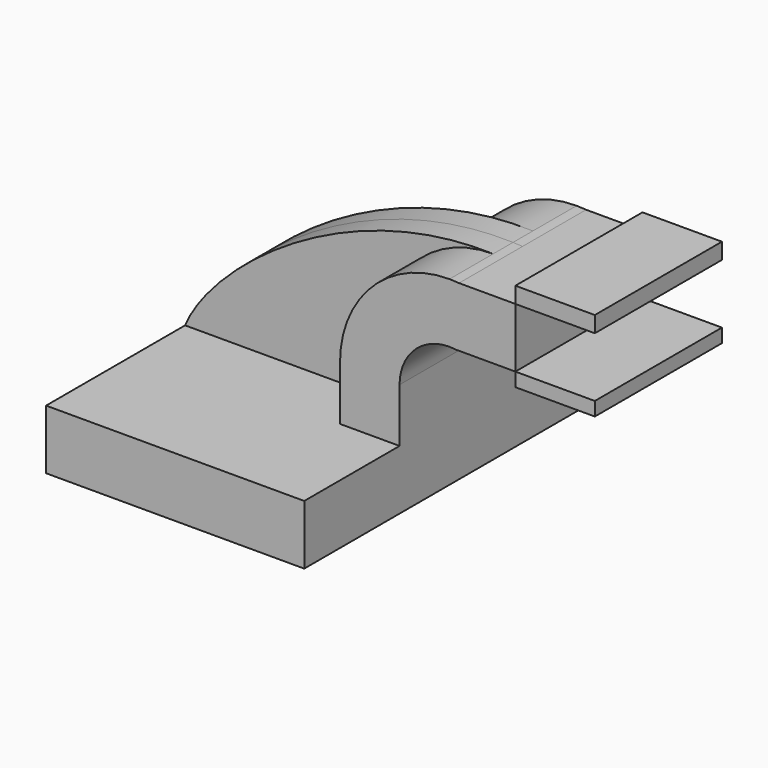
from build123d import *

# Parameters (mm, degrees)
F1_DEPTH = 63.5
F2_DEPTH = 25.4
F0_W     = 25.4
F0_H     = 4.3919570744
F3_DEPTH = 7.9375


with BuildPart() as f1:
    # F0 (on Front) → F1 (new body, symmetric)
    with BuildSketch(Plane.XZ):
        Polygon((22.225, 9.525), (-41.275, 9.525), (-41.275, -9.525), (41.275, -9.525), (41.275, 9.525), align=None)
    extrude(amount=F1_DEPTH, both=True)

    # F0 (on Front) → F2 (join, symmetric)
    with BuildSketch(Plane.XZ):
        with BuildLine():
            Line((22.225, 26.757080531), (22.225, 9.525))
            Line((22.225, 9.525), (41.275, 9.525))
            Line((41.275, 9.525), (41.275, 26.757080531))
            ThreePointArc((41.275, 26.757080531), (46.6952089645, 38.7033338936), (59.2545866966, 42.4919570744))
            Line((59.2545866966, 42.4919570744), (78.3045866966, 42.4919570744))
            Line((78.3045866966, 42.4919570744), (78.3045866966, 61.5419570744))
            Line((78.3045866966, 61.5419570744), (60.2753781947, 61.5419570744))
            add(Edge.make_bspline(
                [(57.2342659347, 61.6819788738), (58.2454948409, 61.6509513635), (59.2592866737, 61.6044274591), (60.2753781947, 61.5419570744)],
                knots=[111.7420916137, 111.7420916137, 111.7420916137, 111.7420916137, 114.0975159009, 114.0975159009, 114.0975159009, 114.0975159009], degree=3))
            ThreePointArc((57.2342659347, 61.6819788738), (32.4841061663, 51.4825594219), (22.225, 26.757080531))
        make_face()
    extrude(amount=F2_DEPTH, both=True)

    # F0 (on Front) → F3 (join, symmetric)
    with BuildSketch(Plane.XZ):
        with BuildLine():
            add(Edge.make_bspline(
                [(-41.275, 9.525), (-32.943705628, 29.7499467941), (9.2612388695, 63.1539340156), (57.2342659347, 61.6819788738)],
                knots=[0, 0, 0, 0, 111.7420916137, 111.7420916137, 111.7420916137, 111.7420916137], degree=3))
            Line((-41.275, 9.525), (22.225, 9.525))
            Line((22.225, 9.525), (22.225, 26.757080531))
            ThreePointArc((22.225, 26.757080531), (32.4841061663, 51.4825594219), (57.2342659347, 61.6819788738))
        make_face()
    extrude(amount=F3_DEPTH, both=True)


with BuildPart() as f2:
    # F0 (on Front) → F2, piece 2 (new body, symmetric)
    with BuildSketch(Plane.XZ):
        Polygon((78.3045866966, 66.675), (78.3045866966, 61.5419570744), (78.4352758357, 61.5419570744), (103.7045866966, 61.5419570744), (103.7045866966, 66.675), align=None)
    extrude(amount=F2_DEPTH, both=True)


with BuildPart() as f2b:
    # F0 (on Front) → F2, piece 3 (new body, symmetric)
    with BuildSketch(Plane.XZ):
        with Locations((91.0045866966, 40.2959785372)):
            Rectangle(F0_W, F0_H)
    extrude(amount=F2_DEPTH, both=True)


solid = Compound([f1.part, f2.part, f2b.part])
